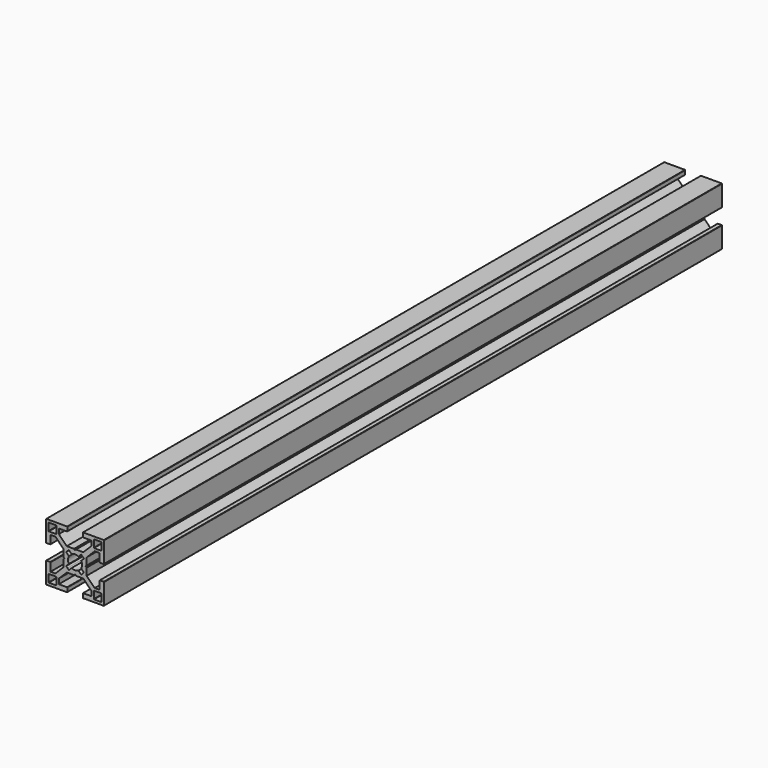
from build123d import *

# Parameters (mm, degrees)
F0_W     = 4
F0_H     = 4
F1_DEPTH = 400
F2_R     = 0.2


# Not quite as in the source:
# - ends of sketch curves that miss each other by under 0.0002 mm in the source are joined


with BuildPart() as f1:
    # F0 (on Front) → F1 (new body)
    with BuildSketch(Plane.XZ):
        Polygon((-4, 12.7), (-4, 15), (-15, 15), (-15, 4), (-12.7, 4), (-12.7, 8.4000005318), (-10.2000002146, 8.4000002226), (-5.9999986286, 4.1999975978), (-5.9999986286, 0.5), (-5.4999986286, 0), (-5.9999986286, -0.5), (-5.9999986286, -4.1999975978), (-10.2000002146, -8.4000002226), (-12.7, -8.4000005401), (-12.7, -4), (-15, -4), (-15, -15), (-4, -15), (-4, -12.7), (-8.4, -12.7), (-8.4, -10.1349351573), (-4.265066287, -6.0000004215), (-0.5, -6.0000004215), (0, -5.5000004215), (0.5, -6.0000004215), (4.265066287, -6.0000004215), (8.4, -10.1349351573), (8.4, -12.7), (4, -12.7), (4, -15), (15, -15), (15, -4), (12.7, -4), (12.7, -8.4000005318), (10.2000002146, -8.4000002143), (5.9999986286, -4.1999975978), (5.9999986286, -0.5), (5.4999986286, 0), (5.9999986286, 0.5), (5.9999986286, 4.1999975978), (10.2000002146, 8.4000002226), (12.7, 8.4000005318), (12.7, 4), (15, 4), (15, 15), (4, 15), (4, 12.7), (8.4, 12.7), (8.4, 10.1349351573), (4.265066287, 6.0000004215), (0.5, 6.0000004215), (0, 5.5000004215), (-0.5, 6.0000004215), (-4.265066287, 6.0000004215), (-8.4, 10.1349351573), (-8.4, 12.7), align=None)
        with Locations((-11.7, -11.7000005318)):
            Rectangle(F0_W, F0_H, mode=Mode.SUBTRACT)
        with Locations((11.7, -11.7000005318)):
            Rectangle(F0_W, F0_H, mode=Mode.SUBTRACT)
        with BuildLine():
            Line((-3.1892931549, 1.7750800467), (-4.6035065879, 3.1892937385))
            Line((-4.6035065879, 3.1892937385), (-3.896399742, 3.896400455))
            Line((-3.896399742, 3.896400455), (-3.1892928961, 4.6035071715))
            Line((-3.1892928961, 4.6035071715), (-1.7750794631, 3.1892934797))
            ThreePointArc((-1.7750794631, 3.1892934797), (-5.13e-08, 3.6466421089), (1.7750793605, 3.1892934797))
            Line((1.7750793605, 3.1892934797), (3.1892927707, 4.6035071942))
            Line((3.1892927707, 4.6035071942), (3.896399628, 3.8964004891))
            Line((3.896399628, 3.8964004891), (4.6035064852, 3.189293784))
            Line((4.6035064852, 3.189293784), (3.189293075, 1.7750800695))
            ThreePointArc((3.189293075, 1.7750800695), (3.6502008105, 3.145e-07), (3.189293075, -1.7750794404))
            Line((3.189293075, -1.7750794404), (4.6035060628, -3.1892944964))
            Line((4.6035060628, -3.1892944964), (3.8964005729, -3.8963996238))
            Line((3.8964005729, -3.8963996238), (3.1892938779, -4.6035064911))
            Line((3.1892938779, -4.6035064911), (1.775078938, -3.189293772))
            ThreePointArc((1.775078938, -3.189293772), (8.169e-07, -3.6522284465), (-1.775078938, -3.189293772))
            Line((-1.775078938, -3.189293772), (-3.1892921382, -4.6035076966))
            Line((-3.1892921382, -4.6035076966), (-3.8964003567, -3.8964000069))
            Line((-3.8964003567, -3.8964000069), (-4.6035070554, -3.1892931432))
            Line((-4.6035070554, -3.1892931432), (-3.1892931549, -1.7750794631))
            ThreePointArc((-3.1892931549, -1.7750794631), (-3.6388745209, 2.918e-07), (-3.1892931549, 1.7750800467))
        make_face(mode=Mode.SUBTRACT)
        with Locations((-11.7, 11.7000005318)):
            Rectangle(F0_W, F0_H, mode=Mode.SUBTRACT)
        with Locations((11.7, 11.7000005318)):
            Rectangle(F0_W, F0_H, mode=Mode.SUBTRACT)
    extrude(amount=F1_DEPTH)

    # F2
    f2_edges = [f1.edges().sort_by_distance(p)[0] for p in [
        (-4, -200, 15),
        (4, -200, 15),
        (-15, -200, 15),
        (15, -200, 15),
        (-12.7, -200, 4),
        (-15, -200, 4),
        (-15, -200, -4),
        (-15, -200, -15),
        (-4, -200, -15),
        (-4, -200, -12.7),
        (-12.7, -200, -4),
        (4, -200, -15),
        (15, -200, -15),
        (12.7, -200, -4),
        (12.7, -200, 4),
        (15, -200, -4),
        (15, -200, 4),
        (-4, -200, 12.7),
        (4, -200, -12.7),
        (4, -200, 12.7),
        (9.7, -200, 13.700001),
        (-13.7, -200, 13.700001),
        (-13.7, -200, -9.700001),
        (9.7, -200, -9.700001),
        (-9.7, -200, 9.700001),
        (-9.7, -200, -13.700001),
        (13.7, -200, -13.700001),
        (13.7, -200, 9.700001),
        (13.7, -200, 13.700001),
        (-9.7, -200, 13.700001),
        (-9.7, -200, -9.700001),
        (13.7, -200, -9.700001),
        (9.7, -200, 9.700001),
        (-13.7, -200, 9.700001),
        (9.7, -200, -13.700001),
        (-13.7, -200, -13.700001),
    ]]
    fillet(f2_edges, radius=F2_R)


solid = f1.part
